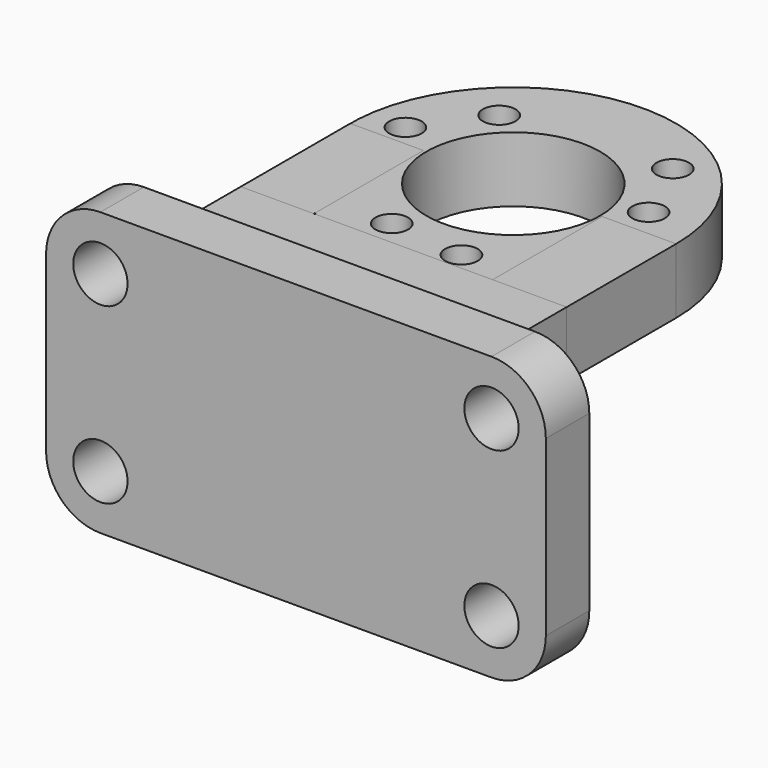
from build123d import *

# Parameters (mm, degrees)
F0_R     = 19.05
F0_R_2   = 1.905
F0_R_3   = 10.16
F1_DEPTH = 7.62
F2_R     = 3.175
F3_DEPTH = 6.35
F4_W     = 38.1
F4_H     = 7.62
F5_DEPTH = 9.398
F6_W     = 8.5519130781
F6_H     = 7.62
F7_DEPTH = 16.002
F6_W_2   = 8.6616750315


# Not quite as in the source:
# - a feature names something its author has since deleted; it is built from what else it names


with BuildPart() as f1:
    # F0 (on Top) → F1 (new body)
    with BuildSketch(Plane.XY):
        with Locations((0, 25.4)):
            Circle(F0_R)
        with Locations((-3.7385604232, 12.3184441793)):
            Circle(F0_R_2, mode=Mode.SUBTRACT)
        with Locations((5.1086041234, 11.4467908741)):
            Circle(F0_R_2, mode=Mode.SUBTRACT)
        with Locations((-14.6401597077, 27.9407882108)):
            Circle(F0_R_2, mode=Mode.SUBTRACT)
        with Locations((-9.4539924163, 35.1612984993)):
            Circle(F0_R_2, mode=Mode.SUBTRACT)
        with Locations((0, 25.4)):
            Circle(F0_R_3, mode=Mode.SUBTRACT)
        with Locations((13.1818417669, 28.7015100533)):
            Circle(F0_R_2, mode=Mode.SUBTRACT)
        with Locations((9.525, 36.8045717149)):
            Circle(F0_R_2, mode=Mode.SUBTRACT)
    extrude(amount=F1_DEPTH)


with BuildPart() as f3:
    # F2 (on Front) → F3 (new body)
    with BuildSketch(Plane.XZ):
        with BuildLine():
            Line((29.2099922622, -16.5000868889), (29.21, 3.8099987387))
            ThreePointArc((29.21, 3.8099987387), (27.3501285065, 8.3001276146), (22.86, 10.16))
            Line((22.86, 10.16), (-22.86, 10.16))
            ThreePointArc((-22.86, 10.16), (-27.3501280662, 8.3001280549), (-29.21, 3.8099999839))
            Line((-29.21, 3.8099999839), (-29.2099999486, -16.51))
            ThreePointArc((-29.2099999486, -16.51), (-27.3505815493, -21.0009571859), (-22.86, -22.8612825818))
            Line((-22.86, -22.8612825818), (22.86, -22.86))
            ThreePointArc((22.86, -22.86), (27.3536315078, -20.9966218776), (29.2099922622, -16.5000868889))
        make_face()
        with Locations((-22.86, -16.51)):
            Circle(F2_R, mode=Mode.SUBTRACT)
        with Locations((22.86, -16.5000868889)):
            Circle(F2_R, mode=Mode.SUBTRACT)
        with Locations((-22.86, 3.81)):
            Circle(F2_R, mode=Mode.SUBTRACT)
        with Locations((22.86, 3.8099987387)):
            Circle(F2_R, mode=Mode.SUBTRACT)
    extrude(amount=F3_DEPTH)


with BuildPart() as f5:
    # F4 (on face) → F5 (new body)
    with BuildSketch(Plane(origin=(0, 0, 0), x_dir=(-1, 0, 0), z_dir=(0, 1, 0))):
        with Locations((0, 3.81)):
            Rectangle(F4_W, F4_H)
    extrude(amount=F5_DEPTH)


with BuildPart() as f7:
    # F6 (on face) → F7 (new body)
    with BuildSketch(Plane(origin=(0, 9.398, 0), x_dir=(-1, 0, 0), z_dir=(0, 1, 0))):
        with Locations((14.7740434609, 3.81)):
            Rectangle(F6_W, F6_H)
    extrude(amount=F7_DEPTH)


with BuildPart() as f7b:
    # F6 (on face) → F7, piece 2 (new body)
    with BuildSketch(Plane(origin=(0, 9.398, 0), x_dir=(-1, 0, 0), z_dir=(0, 1, 0))):
        with Locations((-14.7191624843, 3.81)):
            Rectangle(F6_W_2, F6_H)
    extrude(amount=F7_DEPTH)


solid = Compound([f1.part, f3.part, f5.part, f7.part, f7b.part])
